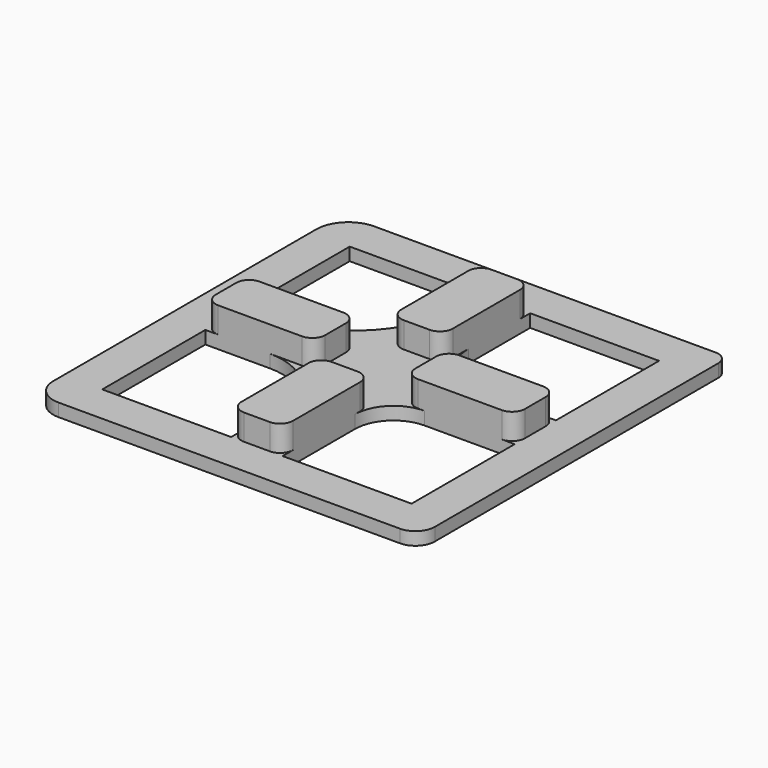
from build123d import *

# Parameters (mm, degrees)
F1_DEPTH     = 2
F3_DEPTH     = 4
F4_TEXT_SIZE = 4.1666666667
F5_DEPTH     = 0.5


# Not quite as in the source:
# - Text() gives the source's letters only with a copy of the font that has no kerning and outlines rounded to 1/6400 em; it was checked with that copy


with BuildPart() as f1:
    # F0 (on Top) → F1 (new body)
    with BuildSketch(Plane.XY):
        with BuildLine():
            ThreePointArc((0, 4), (1.1715728753, 1.1715728753), (4, 0))
            Line((4, 0), (57, 0))
            ThreePointArc((57, 0), (59.1213203436, 0.8786796564), (60, 3))
            Line((60, 3), (60, 58))
            ThreePointArc((60, 58), (59.4142135624, 59.4142135624), (58, 60))
            Line((58, 60), (5, 60))
            ThreePointArc((5, 60), (1.4644660941, 58.5355339059), (0, 55))
            Line((0, 55), (0, 4))
        make_face()
        with BuildLine():
            Line((26, 6), (6, 6))
            Line((6, 6), (6, 26))
            Line((6, 26), (16, 26))
            ThreePointArc((16, 26), (23.0710678119, 23.0710678119), (26, 16))
            Line((26, 16), (26, 6))
        make_face(mode=Mode.SUBTRACT)
        with BuildLine():
            Line((54, 26), (54, 6))
            Line((54, 6), (34, 6))
            Line((34, 6), (34, 20))
            ThreePointArc((34, 20), (35.7573593129, 24.2426406871), (40, 26))
            Line((40, 26), (54, 26))
        make_face(mode=Mode.SUBTRACT)
        with BuildLine():
            Line((6, 34), (6, 54))
            Line((6, 54), (26, 54))
            Line((26, 54), (26, 49))
            ThreePointArc((26, 49), (21.6066017178, 38.3933982822), (11, 34))
            Line((11, 34), (6, 34))
        make_face(mode=Mode.SUBTRACT)
        with BuildLine():
            Line((34, 54), (54, 54))
            Line((54, 54), (54, 34))
            Line((54, 34), (42, 34))
            ThreePointArc((42, 34), (36.3431457505, 36.3431457505), (34, 42))
            Line((34, 42), (34, 54))
        make_face(mode=Mode.SUBTRACT)
    extrude(amount=F1_DEPTH)

    # F2 (on face) → F3 (join)
    with BuildSketch(Plane.XY.offset(2)):
        with BuildLine():
            ThreePointArc((6, 28), (6.5857864376, 26.5857864376), (8, 26))
            Line((8, 26), (21, 26))
            ThreePointArc((21, 26), (22.4142135624, 26.5857864376), (23, 28))
            Line((23, 28), (23, 32))
            ThreePointArc((23, 32), (22.4142135624, 33.4142135624), (21, 34))
            Line((21, 34), (8, 34))
            ThreePointArc((8, 34), (6.5857864376, 33.4142135624), (6, 32))
            Line((6, 32), (6, 28))
        make_face()
        with BuildLine():
            ThreePointArc((34, 52), (33.4142135624, 53.4142135624), (32, 54))
            Line((32, 54), (28, 54))
            ThreePointArc((28, 54), (26.5857864376, 53.4142135624), (26, 52))
            Line((26, 52), (26, 39))
            ThreePointArc((26, 39), (26.5857864376, 37.5857864376), (28, 37))
            Line((28, 37), (32, 37))
            ThreePointArc((32, 37), (33.4142135624, 37.5857864376), (34, 39))
            Line((34, 39), (34, 52))
        make_face()
        with BuildLine():
            Line((28, 6), (32, 6))
            ThreePointArc((32, 6), (33.4142135624, 6.5857864376), (34, 8))
            Line((34, 8), (34, 21))
            ThreePointArc((34, 21), (33.4142135624, 22.4142135624), (32, 23))
            Line((32, 23), (28, 23))
            ThreePointArc((28, 23), (26.5857864376, 22.4142135624), (26, 21))
            Line((26, 21), (26, 8))
            ThreePointArc((26, 8), (26.5857864376, 6.5857864376), (28, 6))
        make_face()
        with BuildLine():
            Line((39, 26), (52, 26))
            ThreePointArc((52, 26), (53.4142135624, 26.5857864376), (54, 28))
            Line((54, 28), (54, 32))
            ThreePointArc((54, 32), (53.4142135624, 33.4142135624), (52, 34))
            Line((52, 34), (39, 34))
            ThreePointArc((39, 34), (37.5857864376, 33.4142135624), (37, 32))
            Line((37, 32), (37, 28))
            ThreePointArc((37, 28), (37.5857864376, 26.5857864376), (39, 26))
        make_face()
    extrude(amount=F3_DEPTH)

    # F4 (on face) → F5 (cut)
    with BuildSketch(Plane(origin=(0, 0, 0), x_dir=(1, 0, 0), z_dir=(0, 0, -1))):
        with Locations((32.6915619713, -27.9229979022)):
            Text('6', F4_TEXT_SIZE, font='Open Sans', font_style=FontStyle.BOLD, text_align=(TextAlign.LEFT, TextAlign.BOTTOM))
        with Locations((23.6467555437, -26.6205872509)):
            Text('10', F4_TEXT_SIZE, font='Open Sans', font_style=FontStyle.BOLD, text_align=(TextAlign.LEFT, TextAlign.BOTTOM))
        with Locations((22.4439650205, -37.634538022)):
            Text('15', F4_TEXT_SIZE, font='Open Sans', font_style=FontStyle.BOLD, text_align=(TextAlign.LEFT, TextAlign.BOTTOM))
        with Locations((33.1588822827, -35.8197946176)):
            Text('8', F4_TEXT_SIZE, font='Open Sans', font_style=FontStyle.BOLD, text_align=(TextAlign.LEFT, TextAlign.BOTTOM))
        with Locations((2.2296088711, -5.1673713774)):
            Text('4', F4_TEXT_SIZE, font='Open Sans', font_style=FontStyle.BOLD, text_align=(TextAlign.LEFT, TextAlign.BOTTOM))
        with Locations((2.7205110481, -57.8290102491)):
            Text('5', F4_TEXT_SIZE, font='Open Sans', font_style=FontStyle.BOLD, text_align=(TextAlign.LEFT, TextAlign.BOTTOM))
        with Locations((55.4309764371, -5.0258832695)):
            Text('3', F4_TEXT_SIZE, font='Open Sans', font_style=FontStyle.BOLD, text_align=(TextAlign.LEFT, TextAlign.BOTTOM))
        with Locations((55.4731853449, -58.2300033811)):
            Text('2', F4_TEXT_SIZE, font='Open Sans', font_style=FontStyle.BOLD, text_align=(TextAlign.LEFT, TextAlign.BOTTOM))
    extrude(amount=-F5_DEPTH, mode=Mode.SUBTRACT)


solid = f1.part
